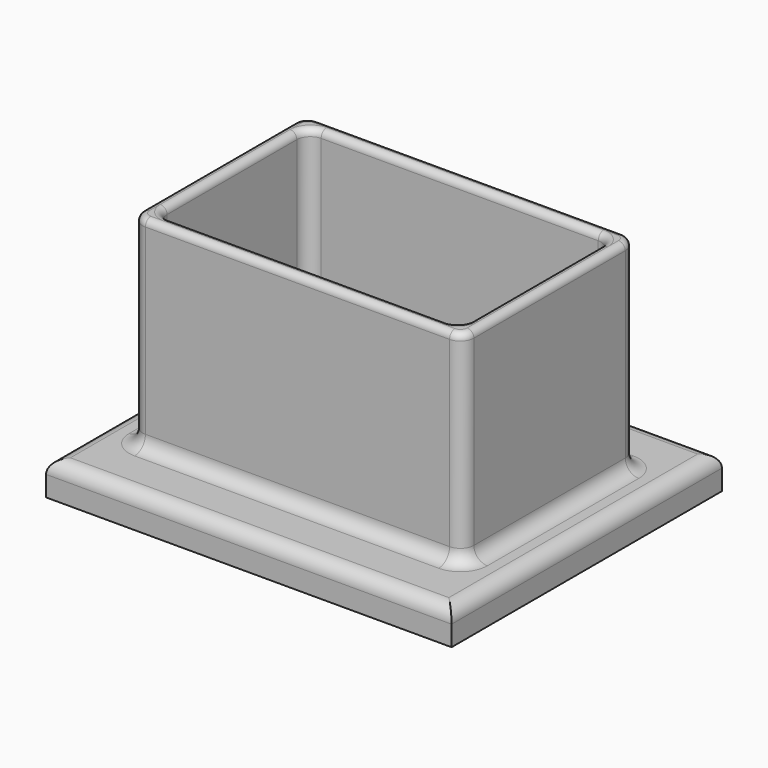
from build123d import *

# Parameters (mm, degrees)
F0_W     = 76.2
F0_H     = 63.5
F1_DEPTH = 6.35
F2_W     = 62.23
F2_H     = 40.64
F2_W_2   = 57.15
F2_H_2   = 35.56
F3_DEPTH = 38.1
F4_R     = 2.54
F5_R     = 1.26999


# Not quite as in the source:
# - a fillet or chamfer is up to 0.001 mm smaller than in the source, because OpenCascade refuses the exact size


with BuildPart() as f1:
    # F0 (on Top) → F1 (new body)
    with BuildSketch(Plane.XY):
        Rectangle(F0_W, F0_H)
    extrude(amount=F1_DEPTH)

    # F2 (on face) → F3 (join)
    with BuildSketch(Plane.XY.offset(6.35)):
        Rectangle(F2_W, F2_H)
        Rectangle(F2_W_2, F2_H_2, mode=Mode.SUBTRACT)
    extrude(amount=F3_DEPTH)

    # F4
    f4_edges = [f1.edges().sort_by_distance(p)[0] for p in [
        (-28.575, 17.78, 25.4),
        (-28.575, -17.78, 25.4),
        (28.575, 17.78, 25.4),
        (28.575, -17.78, 25.4),
        (0, -20.32, 6.35),
        (31.115, 0, 6.35),
        (-31.115, 0, 6.35),
        (0, 20.32, 6.35),
        (0, 31.75, 6.35),
        (-38.1, 0, 6.35),
        (0, -31.75, 6.35),
        (38.1, 0, 6.35),
        (-31.115, -20.32, 25.4),
        (-31.115, 20.32, 25.4),
        (31.115, -20.32, 25.4),
        (31.115, 20.32, 25.4),
    ]]
    fillet(f4_edges, radius=F4_R)

    # F5 (radius 1.27 in the source; OpenCascade refuses exactly that, so slightly less here)
    f5_edges = [f1.edges().sort_by_distance(p)[0] for p in [
        (0, -20.32, 44.45),
        (-30.371051, -19.576051, 44.45),
        (30.371051, -19.576051, 44.45),
        (-31.115, 0, 44.45),
        (31.115, 0, 44.45),
        (-30.371051, 19.576051, 44.45),
        (30.371051, 19.576051, 44.45),
        (0, 20.32, 44.45),
        (28.575, 0, 44.45),
        (27.831051, 17.036051, 44.45),
        (27.831051, -17.036051, 44.45),
        (0, 17.78, 44.45),
        (0, -17.78, 44.45),
        (-27.831051, 17.036051, 44.45),
        (-27.831051, -17.036051, 44.45),
        (-28.575, 0, 44.45),
    ]]
    fillet(f5_edges, radius=F5_R)


solid = f1.part
